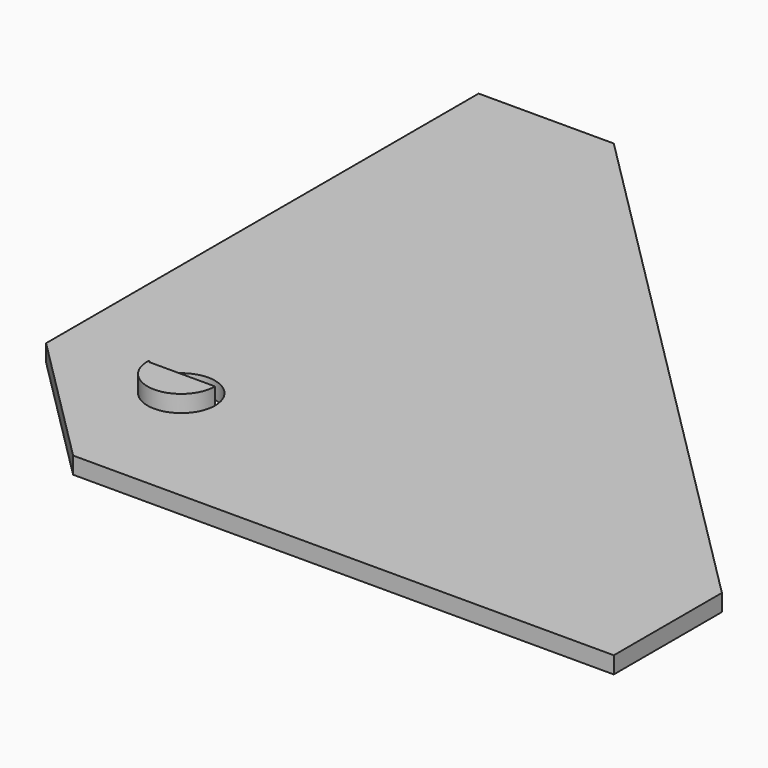
from build123d import *

# Parameters (mm, degrees)
F0_R     = 6.35
F1_DEPTH = 3.175
F3_DEPTH = 3.175


with BuildPart() as f1:
    # F0 (on Top) → F1 (new body)
    with BuildSketch(Plane.XY):
        Polygon((-25.4, 101.6), (-25.4, 0), (0, -25.4), (101.6, -25.4), (101.6, -12.7), (101.6, 0), (0, 101.6), align=None)
        Circle(F0_R, mode=Mode.SUBTRACT)
    extrude(amount=F1_DEPTH)


with BuildPart() as f3:
    # F2 (on face) → F3 (new body)
    with BuildSketch(Plane.XY.offset(3.175)):
        with BuildLine():
            ThreePointArc((-6.3389671749, 0.3741592657), (-0.1871609463, -6.3472411944), (6.35, 0))
            Line((6.35, 0), (-5.9648079092, 0))
            Line((-5.9648079092, 0), (-6.3389671749, 0.3741592657))
        make_face()
    extrude(amount=F3_DEPTH)


solid = Compound([f1.part, f3.part])
